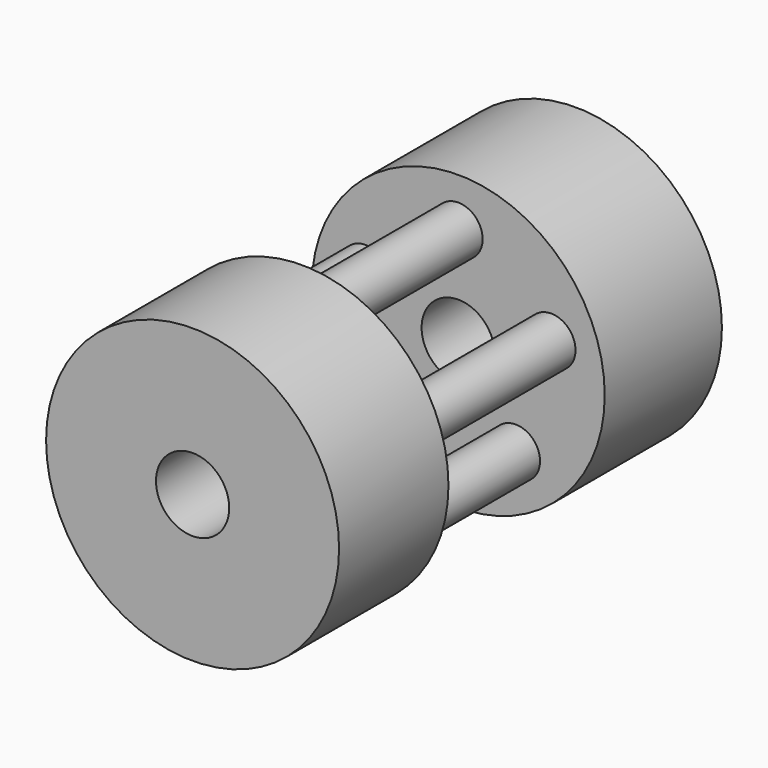
from build123d import *

# Parameters (mm, degrees)
F1_START        = -25.4
F0_R            = 38.1
F1_DEPTH        = 38.1
F2_R            = 6.35
F3_DEPTH        = 50.8
F3_COPIES_COUNT = 5
F4_R            = 38.1
F5_DEPTH        = 35.56
F6_R            = 9.525
F7_DEPTH        = 124.461


# Not quite as in the source:
# - a pattern or mirror of a feature is missing from the dataset's text; its kind, count and spacing are read off the source's solid


with BuildPart() as f1:
    # F0 (on Front) → F1 (new body)
    with BuildSketch(Plane.XZ.offset(F1_START)):
        Circle(F0_R)
    extrude(amount=-F1_DEPTH)

    # F2 (on face) → F3 (join)
    with BuildSketch(Plane.XZ.offset(-25.4)):
        with Locations((0, 25.4)):
            Circle(F2_R)
    f3 = extrude(amount=F3_DEPTH)

    # F3_copies: F3 ×5 about axis
    f3_copies_axis = Axis((0, 0, 0), (0, 1, 0))
    for i in range(1, F3_COPIES_COUNT):
        add(f3.rotate(f3_copies_axis, i * 360 / F3_COPIES_COUNT))

    # F4 (on face) → F5 (join)
    with BuildSketch(Plane.XZ.offset(25.4)):
        Circle(F4_R)
    extrude(amount=F5_DEPTH)

    # F6 (on face) → F7 (cut, through all)
    with BuildSketch(Plane.XZ.offset(60.96)):
        Circle(F6_R)
    extrude(amount=-F7_DEPTH, mode=Mode.SUBTRACT)


solid = f1.part
